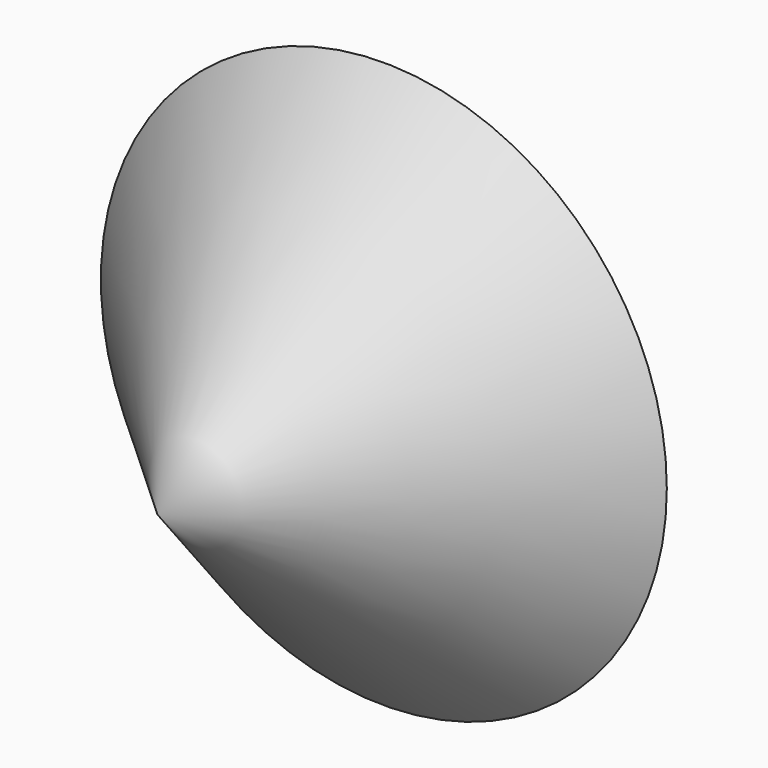
from build123d import *

# Parameters (mm, degrees)
F0_R = 50.543687757


# Not quite as in the source:
# - an extrude whose draft closes it to a point is written as a loft to that point


with BuildPart() as f1:
    # F0 (on Front) → F1 section 0
    with BuildSketch(Plane.XZ, mode=Mode.PRIVATE) as f1_s0:
        Circle(F0_R)
    loft([f1_s0.sketch, Vertex(0, -50.543687757, 0)], ruled=True)


solid = f1.part
